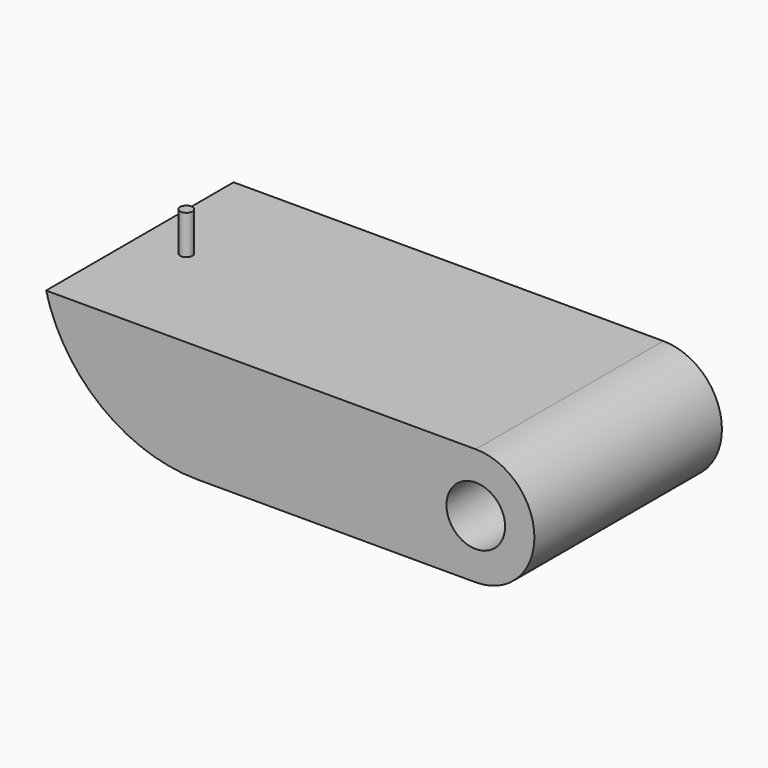
from build123d import *

# Parameters (mm, degrees)
F1_DEPTH    = 38.1
F2_T1_DEPTH = 161.0672212421
F4_D        = 9.525
F5_R        = 1
F6_DEPTH    = 6.35


# Not quite as in the source:
# - a fillet or chamfer that OpenCascade refuses, or shapes differently, is made with other operations: its cross-section is extruded or revolved along the edge and cut away or added


with BuildPart() as f1:
    # F0 (on Front) → F1 (new body)
    with BuildSketch(Plane.XZ):
        with BuildLine():
            Line((37.3479522824, 5.9316984817), (-32.5020477176, 5.9316984817))
            Line((-32.5020477176, 5.9316984817), (-32.5020477176, -13.1183015183))
            Line((-32.5020477176, -13.1183015183), (37.3479522824, -13.1183015183))
            ThreePointArc((37.3479522824, -13.1183015183), (46.8729522824, -3.5933015183), (37.3479522824, 5.9316984817))
        make_face()
    extrude(amount=F1_DEPTH)

    # F2: fillet of radius 25.4 on 1 edges, made by hand

    # F2_s2 → F2_t1 (cut)
    with BuildSketch(Plane.XZ.offset(-61.483610621)):
        with BuildLine():
            ThreePointArc((-32.5020477176, 5.9316984817), (-23.4628633358, -7.7987646603), (-7.9086034692, -13.1183015183))
            Line((-7.9086034692, -13.1183015183), (-32.5020477176, -13.1183015183))
            Line((-32.5020477176, -13.1183015183), (-32.5020477176, 5.9316984817))
        make_face()
    extrude(amount=F2_T1_DEPTH, mode=Mode.SUBTRACT)

    # F4 (through all)
    with Locations(Plane.XZ.offset(38.1)):
        with Locations((37.3479522824, -3.5933015183)):
            Hole(F4_D / 2)

    # F5 (on face) → F6 (join)
    with BuildSketch(Plane.XY.offset(5.9316984817)):
        with Locations((-24.94562231, -19.05)):
            Circle(F5_R)
    extrude(amount=F6_DEPTH)


solid = f1.part
